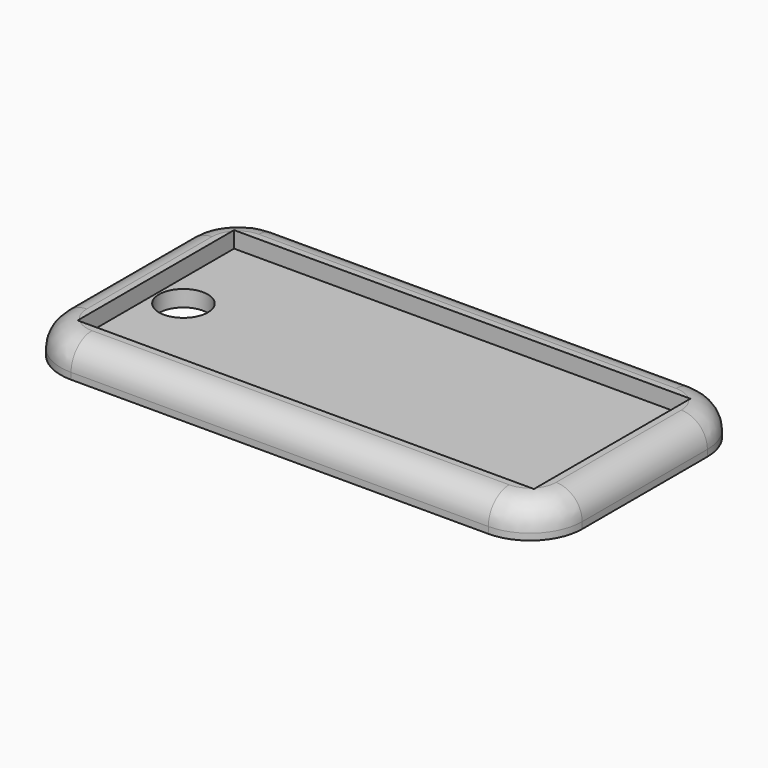
from build123d import *

# Parameters (mm, degrees)
F0_W         = 44.45
F0_H         = 19.05
F0_R         = 2.38125
F1_DEPTH     = 1.5875
F0_W_2       = 50.8
F0_H_2       = 25.4
F2_DEPTH     = 3.175
F3_R         = 5.08
F4_T1_DEPTH  = 40.64
F4_T3_DEPTH  = 15.24
F4_T6_ANGLE  = 90
F4_T8_ANGLE  = 90
F4_T10_ANGLE = 90
F4_T12_ANGLE = 90
F5_TEXT_SIZE = 10.6582743247
F6_DEPTH     = 0.79375


# Not quite as in the source:
# - a fillet or chamfer that OpenCascade refuses, or shapes differently, is made with other operations: its cross-section is extruded or revolved along the edge and cut away or added
# - Text() gives the source's letters only with a copy of the font that has no kerning and outlines rounded to 1/6400 em; it was checked with that copy


with BuildPart() as f1:
    # F0 (on Top) → F1 (new body)
    with BuildSketch(Plane.XY):
        with Locations((25.4, 12.7)):
            Rectangle(F0_W, F0_H)
        with Locations((5.8054751717, 12.7720450982)):
            Circle(F0_R, mode=Mode.SUBTRACT)
    extrude(amount=F1_DEPTH)

    # F0 (on Top) → F2 (join)
    with BuildSketch(Plane.XY):
        with Locations((25.4, 12.7)):
            Rectangle(F0_W_2, F0_H_2)
        with Locations((25.4, 12.7)):
            Rectangle(F0_W, F0_H, mode=Mode.SUBTRACT)
    extrude(amount=F2_DEPTH)

    # F3
    f3_edges = [f1.edges().sort_by_distance(p)[0] for p in [
        (0, 0, 1.5875),
        (50.8, 0, 1.5875),
        (50.8, 25.4, 1.5875),
        (0, 25.4, 1.5875),
    ]]
    fillet(f3_edges, radius=F3_R)

    # F4: fillet of radius 2.54 on 8 edges, made by hand

    # F4_s2 → F4_t1 (cut)
    with BuildSketch(Plane.YZ.offset(5.08)):
        with BuildLine():
            ThreePointArc((0, 0.635), (0.7439487758, 2.4310512242), (2.54, 3.175))
            Line((2.54, 3.175), (0, 3.175))
            Line((0, 3.175), (0, 0.635))
        make_face()
        with BuildLine():
            ThreePointArc((25.4, 0.635), (24.6560512242, 2.4310512242), (22.86, 3.175))
            Line((22.86, 3.175), (25.4, 3.175))
            Line((25.4, 3.175), (25.4, 0.635))
        make_face()
    extrude(amount=F4_T1_DEPTH, mode=Mode.SUBTRACT)

    # F4_s4 → F4_t3 (cut)
    with BuildSketch(Plane.XZ.offset(-20.32)):
        with BuildLine():
            ThreePointArc((0, 0.635), (0.7439487758, 2.4310512242), (2.54, 3.175))
            Line((2.54, 3.175), (0, 3.175))
            Line((0, 3.175), (0, 0.635))
        make_face()
        with BuildLine():
            ThreePointArc((50.8, 0.635), (50.0560512242, 2.4310512242), (48.26, 3.175))
            Line((48.26, 3.175), (50.8, 3.175))
            Line((50.8, 3.175), (50.8, 0.635))
        make_face()
    extrude(amount=F4_T3_DEPTH, mode=Mode.SUBTRACT)

    # F4_s5 → F4_t6 (revolve, cut)
    with BuildSketch(Plane.XZ.offset(-20.32)):
        with BuildLine():
            ThreePointArc((0, 0.635), (0.7439487758, 2.4310512242), (2.54, 3.175))
            Line((2.54, 3.175), (0, 3.175))
            Line((0, 3.175), (0, 0.635))
        make_face()
    revolve(axis=Axis((5.08, 20.32, 3.175), (0, 0, -1)), revolution_arc=F4_T6_ANGLE, mode=Mode.SUBTRACT)

    # F4_s7 → F4_t8 (revolve, cut)
    with BuildSketch(Plane.XZ.offset(-5.08)):
        with BuildLine():
            ThreePointArc((0, 0.635), (0.7439487758, 2.4310512242), (2.54, 3.175))
            Line((2.54, 3.175), (0, 3.175))
            Line((0, 3.175), (0, 0.635))
        make_face()
    revolve(axis=Axis((5.08, 5.08, 3.175), (0, 0, 1)), revolution_arc=F4_T8_ANGLE, mode=Mode.SUBTRACT)

    # F4_s9 → F4_t10 (revolve, cut)
    with BuildSketch(Plane.XZ.offset(-20.32)):
        with BuildLine():
            ThreePointArc((50.8, 0.635), (50.0560512242, 2.4310512242), (48.26, 3.175))
            Line((48.26, 3.175), (50.8, 3.175))
            Line((50.8, 3.175), (50.8, 0.635))
        make_face()
    revolve(axis=Axis((45.72, 20.32, 3.175), (0, 0, 1)), revolution_arc=F4_T10_ANGLE, mode=Mode.SUBTRACT)

    # F4_s11 → F4_t12 (revolve, cut)
    with BuildSketch(Plane.YZ.offset(45.72)):
        with BuildLine():
            ThreePointArc((0, 0.635), (0.7439487758, 2.4310512242), (2.54, 3.175))
            Line((2.54, 3.175), (0, 3.175))
            Line((0, 3.175), (0, 0.635))
        make_face()
    revolve(axis=Axis((45.72, 5.08, 3.175), (0, 0, 1)), revolution_arc=F4_T12_ANGLE, mode=Mode.SUBTRACT)

    # F5 (on Top) → F6 (join)
    with BuildSketch(Plane.XY):
        with Locations((7.9675188012, 8.7904509909)):
            Text('Cassidy', F5_TEXT_SIZE, font='Open Sans', text_align=(TextAlign.LEFT, TextAlign.BOTTOM))
    extrude(amount=F6_DEPTH)


solid = f1.part
